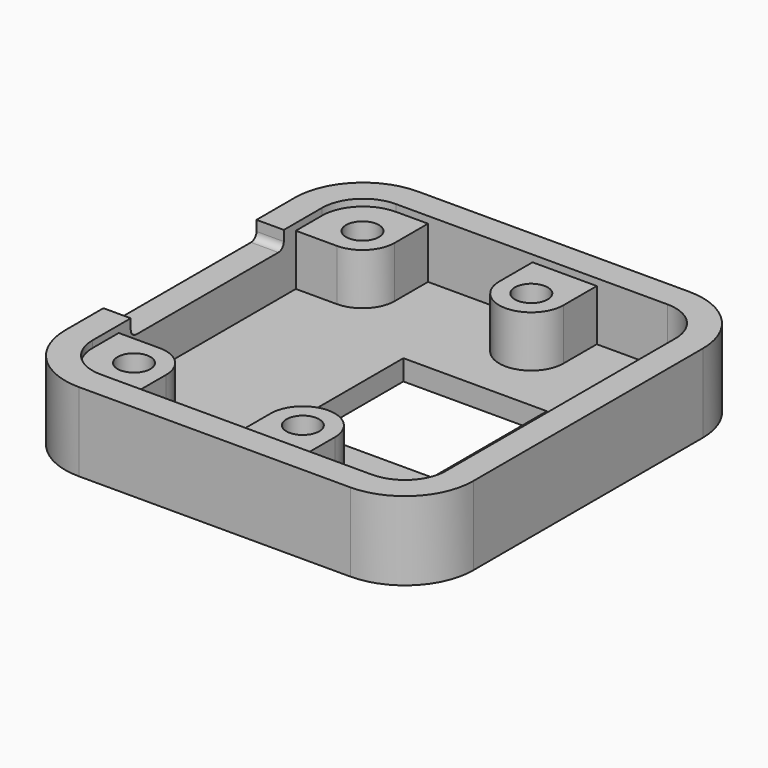
from build123d import *

# Parameters (mm, degrees)
F0_R     = 1.2
F0_W     = 10.5
F0_H     = 10.5
F1_DEPTH = 1.5
F2_DEPTH = 5.25
F3_DEPTH = 5.75
F5_DEPTH = 2


# Not quite as in the source:
# - a feature names something its author has since deleted; it is built from what else it names


with BuildPart() as f1:
    # F0 (on Top) → F1 (new body)
    with BuildSketch(Plane.XY):
        with BuildLine():
            Line((14.9310000289, -10.5), (14.9310000289, 10.5))
            ThreePointArc((14.9310000289, 10.5), (13.4665339264, 14.0355339264), (9.931, 15.5000000289))
            Line((9.931, 15.5000000289), (-9.931, 15.5000000289))
            ThreePointArc((-9.931, 15.5000000289), (-13.4665339264, 14.0355339264), (-14.9310000289, 10.5))
            Line((-14.9310000289, 10.5), (-14.9310000289, -10.5))
            ThreePointArc((-14.9310000289, -10.5), (-13.4665339264, -14.0355339264), (-9.931, -15.5000000289))
            Line((-9.931, -15.5000000289), (9.931, -15.5000000289))
            ThreePointArc((9.931, -15.5000000289), (13.4665339264, -14.0355339264), (14.9310000289, -10.5))
        make_face()
        with BuildLine():
            Line((-9.931, 13.5000000289), (-7.581, 13.5000000289))
            Line((-7.581, 13.5000000289), (0.069, 13.5000000289))
            Line((0.069, 13.5000000289), (4.769, 13.5000000289))
            Line((4.769, 13.5000000289), (9.931, 13.5000000289))
            ThreePointArc((9.931, 13.5000000289), (12.052320364, 12.621320364), (12.9310000289, 10.5))
            Line((12.9310000289, 10.5), (12.9310000289, -10.5))
            ThreePointArc((12.9310000289, -10.5), (12.052320364, -12.621320364), (9.931, -13.5000000289))
            Line((9.931, -13.5000000289), (4.769, -13.5000000289))
            Line((4.769, -13.5000000289), (0.069, -13.5000000289))
            Line((0.069, -13.5000000289), (-7.581, -13.5000000289))
            Line((-7.581, -13.5000000289), (-9.931, -13.5000000289))
            ThreePointArc((-9.931, -13.5000000289), (-12.052320364, -12.621320364), (-12.9310000289, -10.5))
            Line((-12.9310000289, -10.5), (-12.9310000289, -8.1))
            Line((-12.9310000289, -8.1), (-12.9310000289, 8.1))
            Line((-12.9310000289, 8.1), (-12.9310000289, 10.5))
            ThreePointArc((-12.9310000289, 10.5), (-12.052320364, 12.621320364), (-9.931, 13.5000000289))
        make_face(mode=Mode.SUBTRACT)
        with BuildLine():
            ThreePointArc((4.769, -10.45), (2.419, -8.1), (0.069, -10.45))
            ThreePointArc((0.069, -10.45), (2.419, -12.8), (4.769, -10.45))
        make_face()
        with Locations((2.419, -10.45)):
            Circle(F0_R, mode=Mode.SUBTRACT)
        with BuildLine():
            ThreePointArc((4.769, 10.45), (2.419, 12.8), (0.069, 10.45))
            ThreePointArc((0.069, 10.45), (2.419, 8.1), (4.769, 10.45))
        make_face()
        with Locations((2.419, 10.45)):
            Circle(F0_R, mode=Mode.SUBTRACT)
        with BuildLine():
            ThreePointArc((-9.931, 8.1), (-11.5927009358, 12.1117009358), (-7.581, 10.45))
            Line((-7.581, 10.45), (-7.581, 13.5000000289))
            Line((-7.581, 13.5000000289), (-9.931, 13.5000000289))
            ThreePointArc((-9.931, 13.5000000289), (-12.052320364, 12.621320364), (-12.9310000289, 10.5))
            Line((-12.9310000289, 10.5), (-12.9310000289, 8.1))
            Line((-12.9310000289, 8.1), (-9.931, 8.1))
        make_face()
        with BuildLine():
            Line((-9.931, -8.1), (-12.9310000289, -8.1))
            Line((-12.9310000289, -8.1), (-12.9310000289, -10.5))
            ThreePointArc((-12.9310000289, -10.5), (-12.052320364, -12.621320364), (-9.931, -13.5000000289))
            Line((-9.931, -13.5000000289), (-7.581, -13.5000000289))
            Line((-7.581, -13.5000000289), (-7.581, -10.45))
            ThreePointArc((-7.581, -10.45), (-11.5927009358, -12.1117009358), (-9.931, -8.1))
        make_face()
        with BuildLine():
            Line((-7.581, 13.5000000289), (-7.581, 10.45))
            ThreePointArc((-7.581, 10.45), (-8.2692990642, 8.7882990642), (-9.931, 8.1))
            Line((-9.931, 8.1), (-12.9310000289, 8.1))
            Line((-12.9310000289, 8.1), (-12.9310000289, -8.1))
            Line((-12.9310000289, -8.1), (-9.931, -8.1))
            ThreePointArc((-9.931, -8.1), (-8.2692990642, -8.7882990642), (-7.581, -10.45))
            Line((-7.581, -10.45), (-7.581, -13.5000000289))
            Line((-7.581, -13.5000000289), (0.069, -13.5000000289))
            Line((0.069, -13.5000000289), (0.069, -10.45))
            ThreePointArc((0.069, -10.45), (2.419, -8.1), (4.769, -10.45))
            Line((4.769, -10.45), (4.769, -13.5000000289))
            Line((4.769, -13.5000000289), (9.931, -13.5000000289))
            ThreePointArc((9.931, -13.5000000289), (12.052320364, -12.621320364), (12.9310000289, -10.5))
            Line((12.9310000289, -10.5), (12.9310000289, 10.5))
            ThreePointArc((12.9310000289, 10.5), (12.052320364, 12.621320364), (9.931, 13.5000000289))
            Line((9.931, 13.5000000289), (4.769, 13.5000000289))
            Line((4.769, 13.5000000289), (4.769, 10.45))
            ThreePointArc((4.769, 10.45), (2.419, 8.1), (0.069, 10.45))
            Line((0.069, 10.45), (0.069, 13.5000000289))
            Line((0.069, 13.5000000289), (-7.581, 13.5000000289))
        make_face()
        with Locations((2.469, 0)):
            Rectangle(F0_W, F0_H, mode=Mode.SUBTRACT)
        with BuildLine():
            ThreePointArc((-7.581, -10.45), (-8.2692990642, -8.7882990642), (-9.931, -8.1))
            ThreePointArc((-9.931, -8.1), (-11.5927009358, -12.1117009358), (-7.581, -10.45))
        make_face()
        with Locations((-9.931, -10.45)):
            Circle(F0_R, mode=Mode.SUBTRACT)
        with BuildLine():
            Line((0.069, -10.45), (0.069, -13.5000000289))
            Line((0.069, -13.5000000289), (4.769, -13.5000000289))
            Line((4.769, -13.5000000289), (4.769, -10.45))
            ThreePointArc((4.769, -10.45), (2.419, -12.8), (0.069, -10.45))
        make_face()
        with BuildLine():
            ThreePointArc((-9.931, 8.1), (-8.2692990642, 8.7882990642), (-7.581, 10.45))
            ThreePointArc((-7.581, 10.45), (-11.5927009358, 12.1117009358), (-9.931, 8.1))
        make_face()
        with Locations((-9.931, 10.45)):
            Circle(F0_R, mode=Mode.SUBTRACT)
        with BuildLine():
            Line((4.769, 13.5000000289), (0.069, 13.5000000289))
            Line((0.069, 13.5000000289), (0.069, 10.45))
            ThreePointArc((0.069, 10.45), (2.419, 12.8), (4.769, 10.45))
            Line((4.769, 10.45), (4.769, 13.5000000289))
        make_face()
    extrude(amount=F1_DEPTH)

    # F0 (on Top) → F2 (join)
    with BuildSketch(Plane.XY):
        with BuildLine():
            ThreePointArc((-9.931, 8.1), (-11.5927009358, 12.1117009358), (-7.581, 10.45))
            Line((-7.581, 10.45), (-7.581, 13.5000000289))
            Line((-7.581, 13.5000000289), (-9.931, 13.5000000289))
            ThreePointArc((-9.931, 13.5000000289), (-12.052320364, 12.621320364), (-12.9310000289, 10.5))
            Line((-12.9310000289, 10.5), (-12.9310000289, 8.1))
            Line((-12.9310000289, 8.1), (-9.931, 8.1))
        make_face()
        with BuildLine():
            ThreePointArc((-9.931, 8.1), (-8.2692990642, 8.7882990642), (-7.581, 10.45))
            ThreePointArc((-7.581, 10.45), (-11.5927009358, 12.1117009358), (-9.931, 8.1))
        make_face()
        with Locations((-9.931, 10.45)):
            Circle(F0_R, mode=Mode.SUBTRACT)
        with BuildLine():
            ThreePointArc((4.769, 10.45), (2.419, 12.8), (0.069, 10.45))
            ThreePointArc((0.069, 10.45), (2.419, 8.1), (4.769, 10.45))
        make_face()
        with Locations((2.419, 10.45)):
            Circle(F0_R, mode=Mode.SUBTRACT)
        with BuildLine():
            Line((4.769, 13.5000000289), (0.069, 13.5000000289))
            Line((0.069, 13.5000000289), (0.069, 10.45))
            ThreePointArc((0.069, 10.45), (2.419, 12.8), (4.769, 10.45))
            Line((4.769, 10.45), (4.769, 13.5000000289))
        make_face()
        with BuildLine():
            ThreePointArc((4.769, -10.45), (2.419, -8.1), (0.069, -10.45))
            ThreePointArc((0.069, -10.45), (2.419, -12.8), (4.769, -10.45))
        make_face()
        with Locations((2.419, -10.45)):
            Circle(F0_R, mode=Mode.SUBTRACT)
        with BuildLine():
            Line((0.069, -10.45), (0.069, -13.5000000289))
            Line((0.069, -13.5000000289), (4.769, -13.5000000289))
            Line((4.769, -13.5000000289), (4.769, -10.45))
            ThreePointArc((4.769, -10.45), (2.419, -12.8), (0.069, -10.45))
        make_face()
        with BuildLine():
            ThreePointArc((-7.581, -10.45), (-8.2692990642, -8.7882990642), (-9.931, -8.1))
            ThreePointArc((-9.931, -8.1), (-11.5927009358, -12.1117009358), (-7.581, -10.45))
        make_face()
        with Locations((-9.931, -10.45)):
            Circle(F0_R, mode=Mode.SUBTRACT)
        with BuildLine():
            Line((-9.931, -8.1), (-12.9310000289, -8.1))
            Line((-12.9310000289, -8.1), (-12.9310000289, -10.5))
            ThreePointArc((-12.9310000289, -10.5), (-12.052320364, -12.621320364), (-9.931, -13.5000000289))
            Line((-9.931, -13.5000000289), (-7.581, -13.5000000289))
            Line((-7.581, -13.5000000289), (-7.581, -10.45))
            ThreePointArc((-7.581, -10.45), (-11.5927009358, -12.1117009358), (-9.931, -8.1))
        make_face()
    extrude(amount=F2_DEPTH)

    # F0 (on Top) → F3 (join)
    with BuildSketch(Plane.XY):
        with BuildLine():
            Line((14.9310000289, -10.5), (14.9310000289, 10.5))
            ThreePointArc((14.9310000289, 10.5), (13.4665339264, 14.0355339264), (9.931, 15.5000000289))
            Line((9.931, 15.5000000289), (-9.931, 15.5000000289))
            ThreePointArc((-9.931, 15.5000000289), (-13.4665339264, 14.0355339264), (-14.9310000289, 10.5))
            Line((-14.9310000289, 10.5), (-14.9310000289, -10.5))
            ThreePointArc((-14.9310000289, -10.5), (-13.4665339264, -14.0355339264), (-9.931, -15.5000000289))
            Line((-9.931, -15.5000000289), (9.931, -15.5000000289))
            ThreePointArc((9.931, -15.5000000289), (13.4665339264, -14.0355339264), (14.9310000289, -10.5))
        make_face()
        with BuildLine():
            Line((-9.931, 13.5000000289), (-7.581, 13.5000000289))
            Line((-7.581, 13.5000000289), (0.069, 13.5000000289))
            Line((0.069, 13.5000000289), (4.769, 13.5000000289))
            Line((4.769, 13.5000000289), (9.931, 13.5000000289))
            ThreePointArc((9.931, 13.5000000289), (12.052320364, 12.621320364), (12.9310000289, 10.5))
            Line((12.9310000289, 10.5), (12.9310000289, -10.5))
            ThreePointArc((12.9310000289, -10.5), (12.052320364, -12.621320364), (9.931, -13.5000000289))
            Line((9.931, -13.5000000289), (4.769, -13.5000000289))
            Line((4.769, -13.5000000289), (0.069, -13.5000000289))
            Line((0.069, -13.5000000289), (-7.581, -13.5000000289))
            Line((-7.581, -13.5000000289), (-9.931, -13.5000000289))
            ThreePointArc((-9.931, -13.5000000289), (-12.052320364, -12.621320364), (-12.9310000289, -10.5))
            Line((-12.9310000289, -10.5), (-12.9310000289, -8.1))
            Line((-12.9310000289, -8.1), (-12.9310000289, 8.1))
            Line((-12.9310000289, 8.1), (-12.9310000289, 10.5))
            ThreePointArc((-12.9310000289, 10.5), (-12.052320364, 12.621320364), (-9.931, 13.5000000289))
        make_face(mode=Mode.SUBTRACT)
    extrude(amount=F3_DEPTH)

    # F4 (on face) → F5 (cut)
    with BuildSketch(Plane(origin=(-14.9310000289, 0, 0), x_dir=(0, -1, 0), z_dir=(-1, 0, 0))):
        with BuildLine():
            Line((7, 5.75), (-7, 5.75))
            Line((-7, 5.75), (-7, 5))
            ThreePointArc((-7, 5), (-6.8535533906, 4.6464466094), (-6.5, 4.5))
            Line((-6.5, 4.5), (6.5, 4.5))
            ThreePointArc((6.5, 4.5), (6.8535533906, 4.6464466094), (7, 5))
            Line((7, 5), (7, 5.75))
        make_face()
    extrude(amount=-F5_DEPTH, mode=Mode.SUBTRACT)


solid = f1.part
